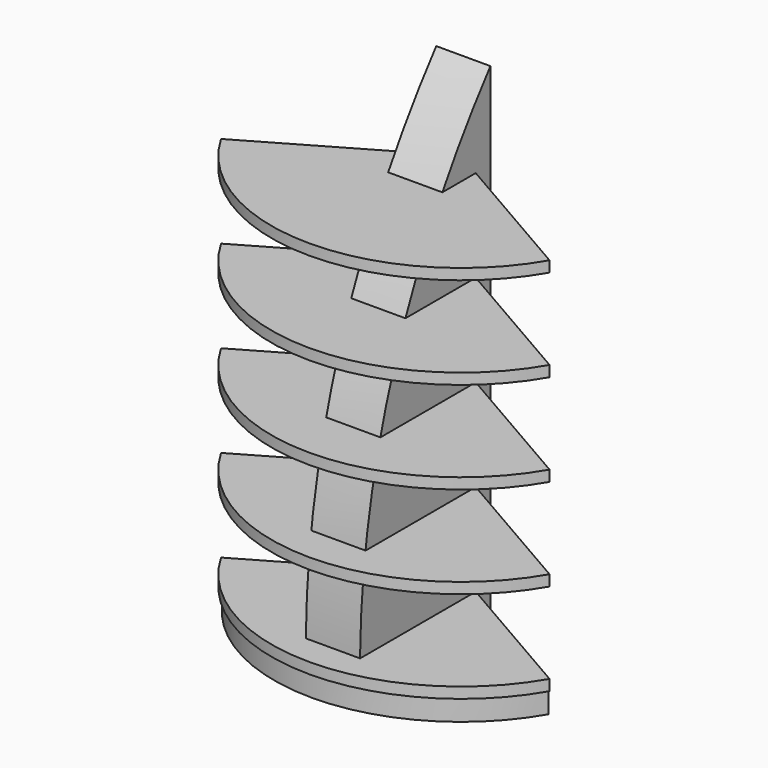
from build123d import *

# Parameters (mm, degrees)
F4_DEPTH      = 200
F6_W          = 690
F6_H          = 80
F7_ANGLE_BACK = 60
F7_ANGLE      = 120
F6_W_2        = 700
F6_H_2        = 40


# Not quite as in the source:
# - a feature of the source that left no trace in its solid (it failed there, or was rolled back) is left out


with BuildPart() as f4:
    # F3 (on Right) → F4 (new body)
    with BuildSketch(Plane.YZ):
        with BuildLine():
            Line((-600, 0), (0, 0))
            Line((0, 0), (0, 1800))
            ThreePointArc((0, 1800), (-461.8112779608, 953.9370926536), (-600, 0))
        make_face()
    extrude(amount=F4_DEPTH)


with BuildPart() as f7:
    # F6 (on offset) → F7 (revolve)
    with BuildSketch(Plane.YZ.offset(100), mode=Mode.PRIVATE) as f7_sk:
        with Locations((-355, 40)):
            Rectangle(F6_W, F6_H)
        Polygon((-700, 80), (-10, 80), (-10, 120), (-710, 120), (-710, 80), align=None)
    revolve(f7_sk.sketch.rotate(Axis((100, -10, 40), (0, 0, 1)), -F7_ANGLE_BACK), axis=Axis((100, -10, 40), (0, 0, 1)), revolution_arc=F7_ANGLE)


with BuildPart() as f7b:
    # F6 (on offset) → F7, piece 2 (revolve)
    with BuildSketch(Plane.YZ.offset(100), mode=Mode.PRIVATE) as f7_sk:
        with Locations((-360, 440)):
            Rectangle(F6_W_2, F6_H_2)
    revolve(f7_sk.sketch.rotate(Axis((100, -10, 40), (0, 0, 1)), -F7_ANGLE_BACK), axis=Axis((100, -10, 40), (0, 0, 1)), revolution_arc=F7_ANGLE)


with BuildPart() as f7c:
    # F6 (on offset) → F7, piece 3 (revolve)
    with BuildSketch(Plane.YZ.offset(100), mode=Mode.PRIVATE) as f7_sk:
        with Locations((-360, 780)):
            Rectangle(F6_W_2, F6_H_2)
    revolve(f7_sk.sketch.rotate(Axis((100, -10, 40), (0, 0, 1)), -F7_ANGLE_BACK), axis=Axis((100, -10, 40), (0, 0, 1)), revolution_arc=F7_ANGLE)


with BuildPart() as f7d:
    # F6 (on offset) → F7, piece 4 (revolve)
    with BuildSketch(Plane.YZ.offset(100), mode=Mode.PRIVATE) as f7_sk:
        with Locations((-360, 1120)):
            Rectangle(F6_W_2, F6_H_2)
    revolve(f7_sk.sketch.rotate(Axis((100, -10, 40), (0, 0, 1)), -F7_ANGLE_BACK), axis=Axis((100, -10, 40), (0, 0, 1)), revolution_arc=F7_ANGLE)


with BuildPart() as f7e:
    # F6 (on offset) → F7, piece 5 (revolve)
    with BuildSketch(Plane.YZ.offset(100), mode=Mode.PRIVATE) as f7_sk:
        with Locations((-360, 1460)):
            Rectangle(F6_W_2, F6_H_2)
    revolve(f7_sk.sketch.rotate(Axis((100, -10, 40), (0, 0, 1)), -F7_ANGLE_BACK), axis=Axis((100, -10, 40), (0, 0, 1)), revolution_arc=F7_ANGLE)


solid = Compound([f4.part, f7.part, f7b.part, f7c.part, f7d.part, f7e.part])
